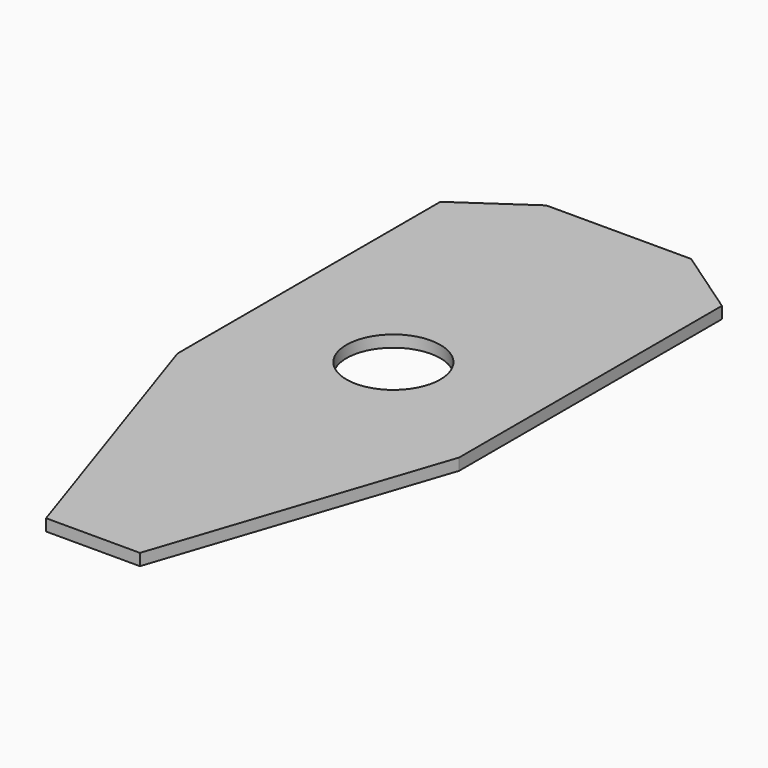
from build123d import *

# Parameters (mm, degrees)
F0_R     = 12.7
F1_DEPTH = 3.175


# Not quite as in the source:
# - a length typed as a fraction of an inch, garbled in the dataset ("3 / 203.2 mm" for 3/8 in), is restored


with BuildPart() as f1:
    # F0 (on Top) → F1 (new body)
    with BuildSketch(Plane.XY):
        Polygon((-38.1, 0), (-12.7, -76.2), (12.7, -76.2), (38.1, 0), (38.1, 50.8), (38.1, 88.9), (19.6133758873, 101.6), (-19.6133758873, 101.6), (-38.1, 88.9), (-38.1, 50.8), align=None)
        with Locations((0, 25.4)):
            Circle(F0_R, mode=Mode.SUBTRACT)
    extrude(amount=-F1_DEPTH)


solid = f1.part
